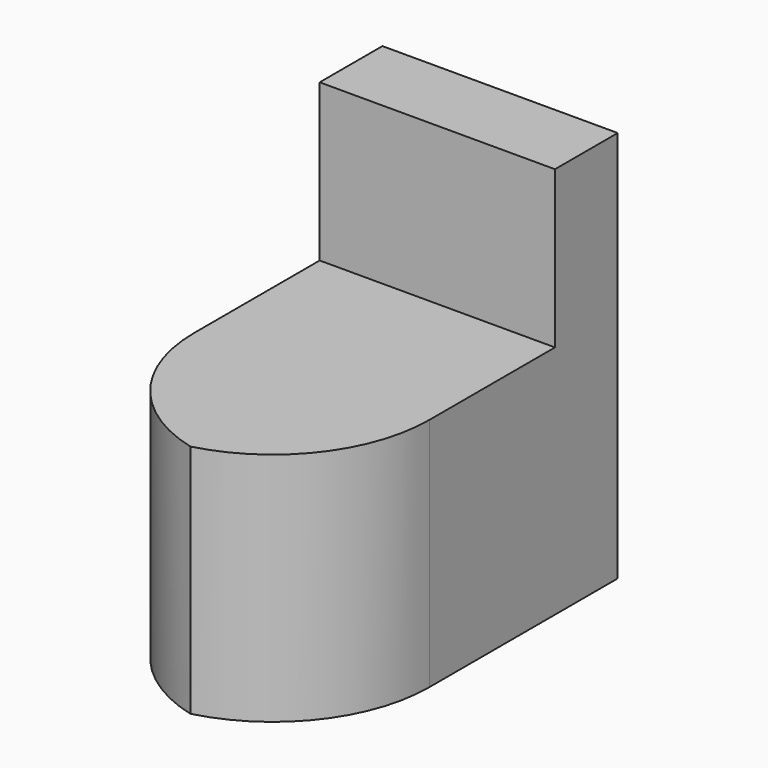
from build123d import *

# Parameters (mm, degrees)
F0_W        = 457.2
F0_H        = 762
F1_DEPTH    = 762
F2_W        = 457.2
F2_H        = 304.8
F3_DEPTH    = 609.6
F4_T1_DEPTH = 1981.2


# Not quite as in the source:
# - a fillet or chamfer that OpenCascade refuses, or shapes differently, is made with other operations: its cross-section is extruded or revolved along the edge and cut away or added


with BuildPart() as f1:
    # F0 (on Front) → F1 (new body)
    with BuildSketch(Plane.XZ):
        Rectangle(F0_W, F0_H)
    extrude(amount=F1_DEPTH)

    # F2 (on face) → F3 (cut)
    with BuildSketch(Plane.XZ.offset(762)):
        with Locations((0, 228.6)):
            Rectangle(F2_W, F2_H)
    extrude(amount=-F3_DEPTH, mode=Mode.SUBTRACT)

    # F4: fillet of radius 304.8 on 2 edges, made by hand

    # F4_s2 → F4_t1 (cut)
    with BuildSketch(Plane.XY.offset(-1143)):
        with BuildLine():
            ThreePointArc((-228.6, -457.2), (-139.3261469057, -672.7261469057), (76.2, -762))
            Line((76.2, -762), (-228.6, -762))
            Line((-228.6, -762), (-228.6, -457.2))
        make_face()
        with BuildLine():
            ThreePointArc((228.6, -457.2), (139.3261469057, -672.7261469057), (-76.2, -762))
            Line((-76.2, -762), (228.6, -762))
            Line((228.6, -762), (228.6, -457.2))
        make_face()
    extrude(amount=F4_T1_DEPTH, mode=Mode.SUBTRACT)


solid = f1.part
